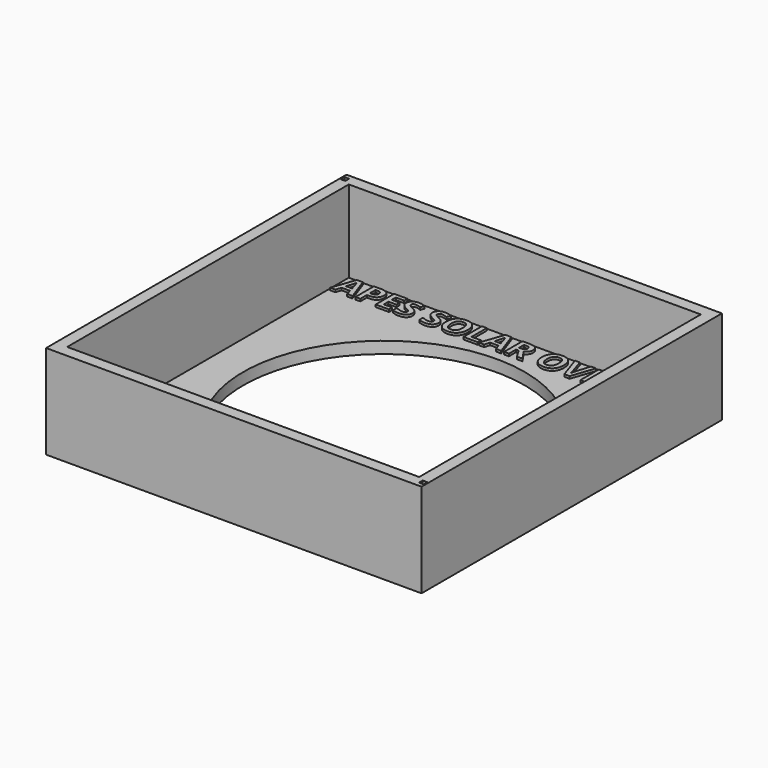
from build123d import *

# Parameters (mm, degrees)
F0_W          = 203.2
F0_H          = 203.2
F1_DEPTH      = 50.8
F2_W          = 190.5
F2_H          = 190.5
F3_DEPTH      = 44.45
F4_R          = 76.2
F5_DEPTH      = 6.604
F6_TEXT_SIZE  = 17.4808936814
F7_DEPTH      = 1.27
F8_W          = 2.54
F8_H          = 2.54
F9_DEPTH      = 5.08
F10_W         = 2.54
F10_H         = 2.54
F11_DEPTH     = 5.08
F12_TEXT_SIZE = 11.5513304334
F13_DEPTH     = 1.27


# Not quite as in the source:
# - Text() gives the source's letters only with a copy of the font that has no kerning and outlines rounded to 1/6400 em; it was checked with that copy


with BuildPart() as f1:
    # F0 (on Top) → F1 (new body)
    with BuildSketch(Plane.XY):
        Rectangle(F0_W, F0_H)
    extrude(amount=F1_DEPTH)

    # F2 (on face) → F3 (cut)
    with BuildSketch(Plane.XY.offset(50.8)):
        Rectangle(F2_W, F2_H)
    extrude(amount=-F3_DEPTH, mode=Mode.SUBTRACT)

    # F4 (on face) → F5 (cut)
    with BuildSketch(Plane.XY.offset(6.35)):
        Circle(F4_R)
    extrude(amount=-F5_DEPTH, mode=Mode.SUBTRACT)

    # F6 (on face) → F7 (join)
    with BuildSketch(Plane.XY.offset(6.35)):
        with Locations((-94.158872962, 81.3175141811)):
            Text("APES SOLAR OVEN 17'", F6_TEXT_SIZE, font='Open Sans', font_style=FontStyle.BOLD, text_align=(TextAlign.LEFT, TextAlign.BOTTOM))
    extrude(amount=F7_DEPTH)

    # F8 (on face) → F9 (cut)
    with BuildSketch(Plane.XY.offset(50.8)):
        with Locations((-99.6696, 98.0948)):
            Rectangle(F8_W, F8_H)
    extrude(amount=-F9_DEPTH, mode=Mode.SUBTRACT)

    # F10 (on face) → F11 (cut)
    with BuildSketch(Plane.XY.offset(50.8)):
        with Locations((99.6696, -98.0948)):
            Rectangle(F10_W, F10_H)
    extrude(amount=-F11_DEPTH, mode=Mode.SUBTRACT)

    # F12 (on face) → F13 (join)
    with BuildSketch(Plane.XY.offset(6.35)):
        with Locations((-92.71, -93.0977868941)):
            Text('MAY ALL WHO ENTER LEAVE BAKED', F12_TEXT_SIZE, font='Open Sans', font_style=FontStyle.BOLDITALIC, text_align=(TextAlign.LEFT, TextAlign.BOTTOM))
    extrude(amount=F13_DEPTH)


solid = f1.part
